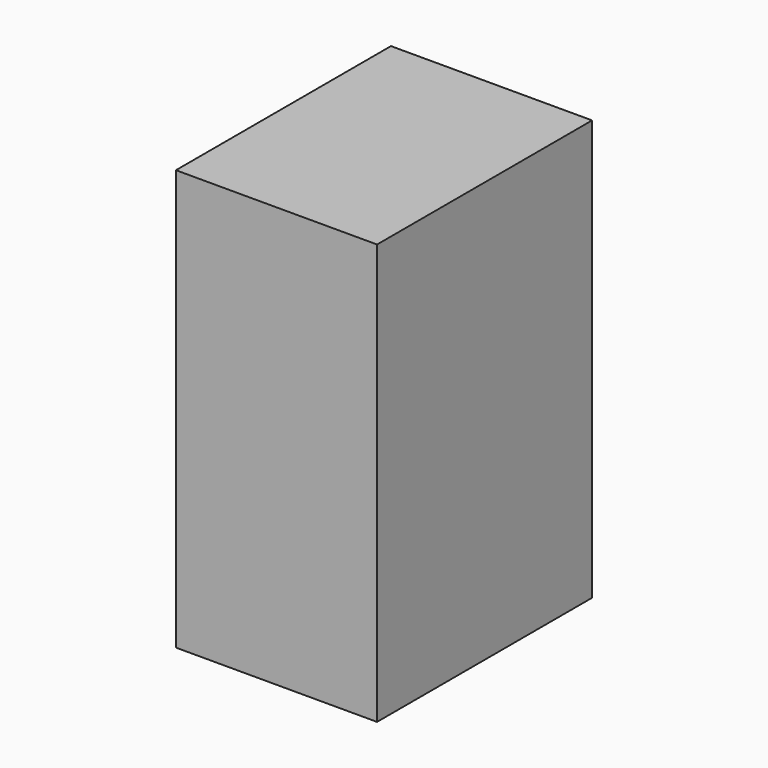
from build123d import *

# Parameters (mm, degrees)
F0_W     = 33.941835165
F0_H     = 53.0750602484
F1_DEPTH = 25.4


# Not quite as in the source:
# - the program builds the solid bodies; features that only make, move or delete a surface that nothing else refers to are left out


with BuildPart() as f1:
    # F0 (on Right) → F1 (new body)
    with BuildSketch(Plane.YZ):
        with Locations((16.9709175825, -2.4021938443)):
            Rectangle(F0_W, F0_H)
    extrude(amount=F1_DEPTH)


solid = f1.part
